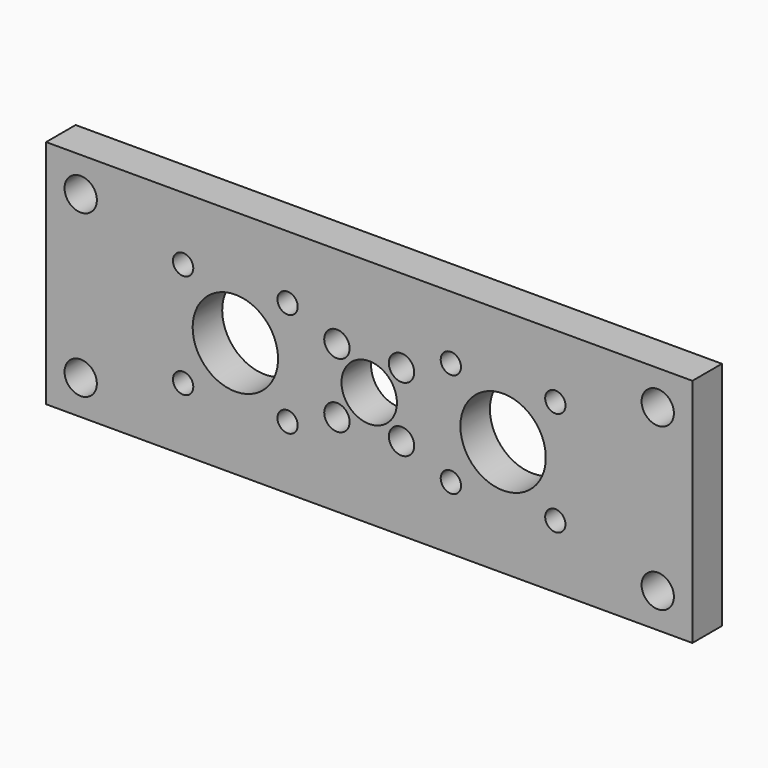
from build123d import *

# Parameters (mm, degrees)
F0_W             = 140
F0_H             = 50
F1_DEPTH         = 8
F3_D             = 12
F4_D             = 5.5
F5_D             = 7
F6_D             = 18.5
F7_D             = 4.4
F7_COPIES_COUNT  = 4
F7_COPIES4_COUNT = 2
F7_COPIES4_PITCH = 62.25753


# Not quite as in the source:
# - a pattern or mirror of a feature is missing from the dataset's text; its kind, count and spacing are read off the source's solid


with BuildPart() as f1:
    # F0 (on Front) → F1 (new body)
    with BuildSketch(Plane.XZ):
        Rectangle(F0_W, F0_H)
    extrude(amount=F1_DEPTH)

    # F3 (through all)
    with Locations(Plane.XZ.offset(8)):
        with Locations((0, 0)):
            Hole(F3_D / 2)

    # F4 (through all)
    with Locations(Plane.XZ.offset(8)):
        with Locations((-7, 7), (-7, -7), (7, -7), (7, 7)):
            Hole(F4_D / 2)

    # F5 (through all)
    with Locations(Plane.XZ.offset(8)):
        with Locations((-62.5, -17.5), (62.5, -17.5), (62.5, 17.5), (-62.5, 17.5)):
            Hole(F5_D / 2)

    # F6 (through all)
    with Locations(Plane.XZ.offset(8)):
        with Locations((-29, 0), (29, 0)):
            Hole(F6_D / 2)

    # F7 (through all)
    with Locations(Plane.XZ.offset(8)):
        with Locations((-40.313708499, 11.313708499)):
            f7 = Hole(F7_D / 2)

    # F7_copies: F7 ×4 about axis
    f7_copies_axis = Axis((-29, 0, 0), (0, 1, 0))
    for i in range(1, F7_COPIES_COUNT):
        add(f7.rotate(f7_copies_axis, i * 360 / F7_COPIES_COUNT), mode=Mode.SUBTRACT)

    # F7_copies1: F7 across plane
    add(f7.mirror(Plane(origin=(0, 0, 0), x_dir=(0, 0, 1), z_dir=(1, 0, 0))), mode=Mode.SUBTRACT)

    # F7_copies2: F7 across plane
    add(f7.mirror(Plane(origin=(-11.313708, 0, 0), x_dir=(0, 0, 1), z_dir=(1, 0, 0))), mode=Mode.SUBTRACT)

    # F7_copies3: F7 across plane
    add(f7.mirror(Plane(origin=(0, 0, 0), x_dir=(0.2702028103, 0, 0.9628034282), z_dir=(0.9628034282, 0, -0.2702028103))), mode=Mode.SUBTRACT)

    # F7_copies4: F7 ×2
    with Locations(*[Vector(0.931614221, 0, -0.3634486803) * (i * F7_COPIES4_PITCH) for i in range(1, F7_COPIES4_COUNT)]):
        add(f7, mode=Mode.SUBTRACT)


solid = f1.part
